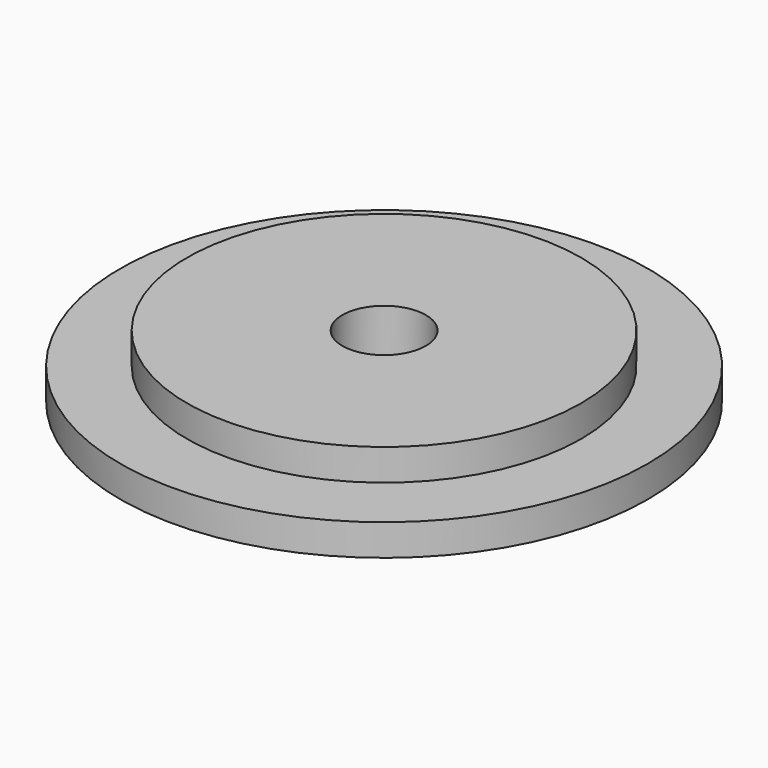
from build123d import *

# Parameters (mm, degrees)
F0_R     = 7.493
F0_R_2   = 1.5875
F1_DEPTH = 1.1938
F2_R     = 10.033
F2_R_2   = 7.493
F2_R_3   = 1.5875
F3_DEPTH = 1.1938


with BuildPart() as f1:
    # F0 (on Top) → F1 (new body)
    with BuildSketch(Plane.XY):
        Circle(F0_R)
        Circle(F0_R_2, mode=Mode.SUBTRACT)
    extrude(amount=F1_DEPTH)

    # F2 (on face) → F3 (join)
    with BuildSketch(Plane(origin=(0, 0, 0), x_dir=(1, 0, 0), z_dir=(0, 0, -1))):
        Circle(F2_R)
        Circle(F2_R_2, mode=Mode.SUBTRACT)
        Circle(F2_R_2)
        Circle(F2_R_3, mode=Mode.SUBTRACT)
    extrude(amount=F3_DEPTH)


solid = f1.part
